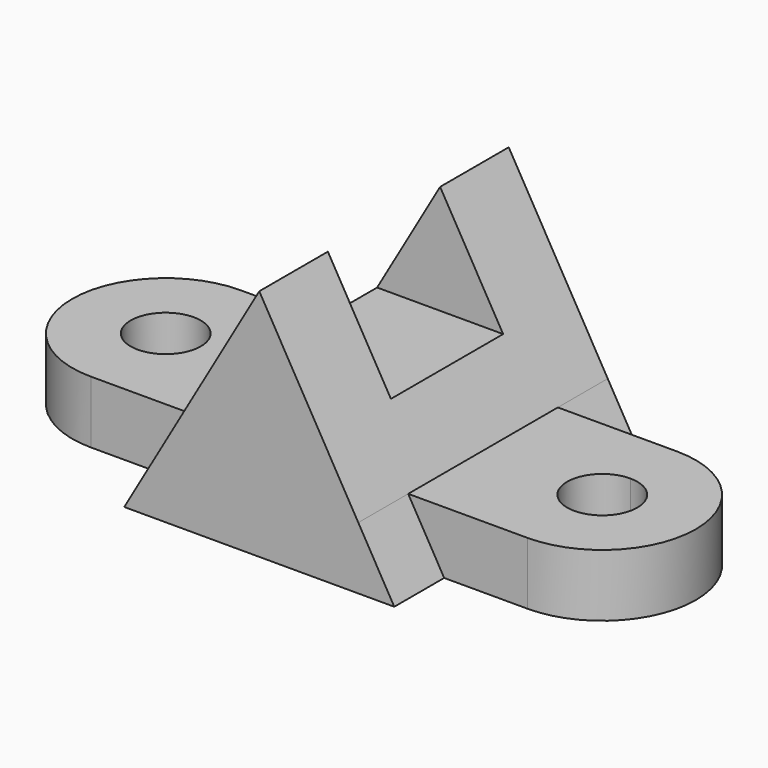
from build123d import *

# Parameters (mm, degrees)
F1_DEPTH = 31.75
F2_DEPTH = 19.05
F5_DEPTH = 12.7
F6_DEPTH = 25.4
F7_DEPTH = 25.4
F8_W     = 40.1893556118
F8_H     = 22.225
F8_W_2   = 32.2620980442
F9_DEPTH = 14.2875


with BuildPart() as f1:
    # F0 (on Front) → F1 (new body, symmetric)
    with BuildSketch(Plane.XZ):
        Polygon((0, 47.625), (0, 12.7), (20.1639581514, 12.7), align=None)
        Polygon((-27.4963065702, 0), (0, 0), (0, 12.7), (-20.1639581514, 12.7), align=None)
        Polygon((0, 12.7), (0, 0), (27.4963065702, 0), (20.1639581514, 12.7), align=None)
        Polygon((-20.1639581514, 12.7), (0, 12.7), (0, 47.625), align=None)
    extrude(amount=F1_DEPTH, both=True)

    # F0 (on Front) → F2 (join, symmetric)
    with BuildSketch(Plane.XZ):
        Polygon((-27.4963065702, 0), (0, 0), (0, 12.7), (-20.1639581514, 12.7), align=None)
        Polygon((0, 12.7), (0, 0), (27.4963065702, 0), (20.1639581514, 12.7), align=None)
        Polygon((-20.1639581514, 12.7), (0, 12.7), (0, 47.625), align=None)
        Polygon((0, 47.625), (0, 12.7), (20.1639581514, 12.7), align=None)
        Polygon((-44.45, 0), (-27.4963065702, 0), (-20.1639581514, 12.7), (-44.45, 12.7), align=None)
        Polygon((20.1639581514, 12.7), (27.4963065702, 0), (44.45, 0), (44.45, 12.7), align=None)
    extrude(amount=F2_DEPTH, both=True)

    # F4 (on face) + F3 (on face) → F5 (join, through all)
    with BuildSketch(Plane.XY.offset(12.7)):
        with BuildLine():
            ThreePointArc((44.45, -19.05), (57.9203841816, -13.4703841816), (63.5, 0))
            ThreePointArc((63.5, 0), (57.9203841816, 13.4703841816), (44.45, 19.05))
            Line((44.45, 19.05), (44.45, 7.14375))
            ThreePointArc((44.45, 7.14375), (49.5013940681, 5.0513940681), (51.59375, 0))
            ThreePointArc((51.59375, 0), (49.5013940681, -5.0513940681), (44.45, -7.14375))
            Line((44.45, -7.14375), (44.45, -19.05))
        make_face()
        with BuildLine():
            Line((44.45, 7.14375), (44.45, 19.05))
            ThreePointArc((44.45, 19.05), (25.4, 0), (44.45, -19.05))
            Line((44.45, -19.05), (44.45, -7.14375))
            ThreePointArc((44.45, -7.14375), (37.30625, 0), (44.45, 7.14375))
        make_face()
    with BuildSketch(Plane.XY.offset(12.7)):
        with BuildLine():
            ThreePointArc((-44.45, -19.05), (-30.9796158184, -13.4703841816), (-25.4, 0))
            ThreePointArc((-25.4, 0), (-30.9796158184, 13.4703841816), (-44.45, 19.05))
            Line((-44.45, 19.05), (-44.45, 7.14375))
            ThreePointArc((-44.45, 7.14375), (-39.3986059319, 5.0513940681), (-37.30625, 0))
            ThreePointArc((-37.30625, 0), (-39.3986059319, -5.0513940681), (-44.45, -7.14375))
            Line((-44.45, -7.14375), (-44.45, -19.05))
        make_face()
        with BuildLine():
            Line((-44.45, 7.14375), (-44.45, 19.05))
            ThreePointArc((-44.45, 19.05), (-63.5, 0), (-44.45, -19.05))
            Line((-44.45, -19.05), (-44.45, -7.14375))
            ThreePointArc((-44.45, -7.14375), (-51.59375, 0), (-44.45, 7.14375))
        make_face()
    extrude(amount=-F5_DEPTH)

    # F3 (on face) → F6 (cut)
    with BuildSketch(Plane.XY.offset(12.7)):
        with BuildLine():
            ThreePointArc((-37.30625, 0), (-39.3986059319, 5.0513940681), (-44.45, 7.14375))
            Line((-44.45, 7.14375), (-44.45, -7.14375))
            ThreePointArc((-44.45, -7.14375), (-39.3986059319, -5.0513940681), (-37.30625, 0))
        make_face()
        with BuildLine():
            Line((-44.45, -7.14375), (-44.45, 7.14375))
            ThreePointArc((-44.45, 7.14375), (-51.59375, 0), (-44.45, -7.14375))
        make_face()
    extrude(amount=-F6_DEPTH, mode=Mode.SUBTRACT)

    # F4 (on face) → F7 (cut)
    with BuildSketch(Plane.XY.offset(12.7)):
        with BuildLine():
            Line((44.45, -7.14375), (44.45, 7.14375))
            ThreePointArc((44.45, 7.14375), (37.30625, 0), (44.45, -7.14375))
        make_face()
    extrude(amount=-F7_DEPTH, mode=Mode.SUBTRACT)

    # F8 (on Front) → F9 (cut, symmetric)
    with BuildSketch(Plane.XZ):
        with Locations((-20.0946778059, 36.5125)):
            Rectangle(F8_W, F8_H)
        with Locations((16.1310490221, 36.5125)):
            Rectangle(F8_W_2, F8_H)
    extrude(amount=F9_DEPTH, both=True, mode=Mode.SUBTRACT)


solid = f1.part
